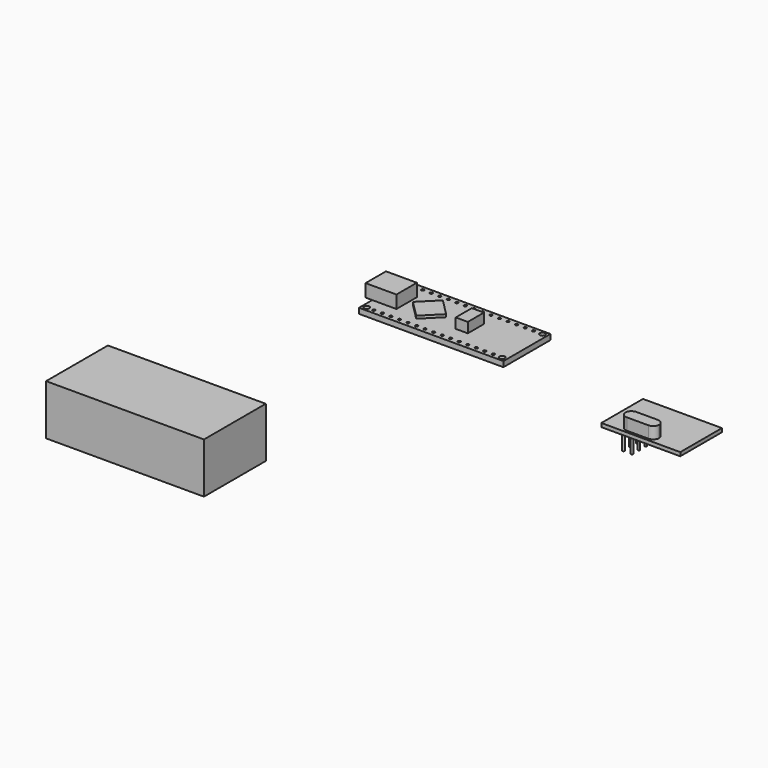
from build123d import *

# Parameters (mm, degrees)
F0_W         = 43
F0_H         = 17.5
F1_DEPTH     = 1.6
F2_R         = 0.8
F3_DEPTH     = 1.6
F4_R         = 0.4
F5_DEPTH     = 1.6
F6_W         = 9.2
F6_H         = 7.6
F7_DEPTH     = 3.8
F9_DEPTH     = 0.8
F10_W        = 3.6
F10_H        = 6
F11_DEPTH    = 3
F12_W        = 23.5
F12_H        = 15.5
F13_DEPTH    = 1.1
F14_W        = 10
F14_H        = 3.5
F15_DEPTH    = 3.5
F16_T1_DEPTH = 8
F17_W        = 2.54
F17_H        = 2.4
F17_H_2      = 0.14
F17_H_3      = 2.54
F18_DEPTH    = 2.6
F19_R        = 0.3
F20_DEPTH    = 5.7
F21_W        = 47
F21_H        = 23
F22_DEPTH    = 15


# Not quite as in the source:
# - a fillet or chamfer that OpenCascade refuses, or shapes differently, is made with other operations: its cross-section is extruded or revolved along the edge and cut away or added


with BuildPart() as f1:
    # F0 (on Top) → F1 (new body)
    with BuildSketch(Plane.XY):
        with Locations((-32.1257647276, 51.5529857576)):
            Rectangle(F0_W, F0_H)
    extrude(amount=F1_DEPTH)

    # F2 (on face) → F3 (cut, through all)
    with BuildSketch(Plane.XY.offset(1.6)):
        with Locations((-52.312482166, 59.0704187174)):
            Circle(F2_R)
        with Locations((-12.012482166, 59.0704187174)):
            Circle(F2_R)
        with Locations((-52.312482166, 44.0704187174)):
            Circle(F2_R)
        with Locations((-12.012482166, 44.0704187174)):
            Circle(F2_R)
    extrude(amount=-F3_DEPTH, mode=Mode.SUBTRACT)

    # F4 (on face) → F5 (cut, through all)
    with BuildSketch(Plane.XY.offset(1.6)):
        with Locations((-50.1963980496, 59.0704187174)):
            Circle(F4_R)
        with Locations((-47.6563980496, 59.0704187174)):
            Circle(F4_R)
        with Locations((-45.1163980496, 59.0704187174)):
            Circle(F4_R)
        with Locations((-42.5763980496, 59.0704187174)):
            Circle(F4_R)
        with Locations((-40.0363980496, 59.0704187174)):
            Circle(F4_R)
        with Locations((-37.4963980496, 59.0704187174)):
            Circle(F4_R)
        with Locations((-34.9563980496, 59.0704187174)):
            Circle(F4_R)
        with Locations((-32.4163980496, 59.0704187174)):
            Circle(F4_R)
        with Locations((-29.8763980496, 59.0704187174)):
            Circle(F4_R)
        with Locations((-27.3363980496, 59.0704187174)):
            Circle(F4_R)
        with Locations((-24.7963980496, 59.0704187174)):
            Circle(F4_R)
        with Locations((-22.2563980496, 59.0704187174)):
            Circle(F4_R)
        with Locations((-19.7163980496, 59.0704187174)):
            Circle(F4_R)
        with Locations((-17.1763980496, 59.0704187174)):
            Circle(F4_R)
        with Locations((-14.6363980496, 59.0704187174)):
            Circle(F4_R)
        with Locations((-50.1963980496, 44.0704187174)):
            Circle(F4_R)
        with Locations((-47.6563980496, 44.0704187174)):
            Circle(F4_R)
        with Locations((-45.1163980496, 44.0704187174)):
            Circle(F4_R)
        with Locations((-42.5763980496, 44.0704187174)):
            Circle(F4_R)
        with Locations((-40.0363980496, 44.0704187174)):
            Circle(F4_R)
        with Locations((-37.4963980496, 44.0704187174)):
            Circle(F4_R)
        with Locations((-34.9563980496, 44.0704187174)):
            Circle(F4_R)
        with Locations((-32.4163980496, 44.0704187174)):
            Circle(F4_R)
        with Locations((-29.8763980496, 44.0704187174)):
            Circle(F4_R)
        with Locations((-27.3363980496, 44.0704187174)):
            Circle(F4_R)
        with Locations((-24.7963980496, 44.0704187174)):
            Circle(F4_R)
        with Locations((-22.2563980496, 44.0704187174)):
            Circle(F4_R)
        with Locations((-19.7163980496, 44.0704187174)):
            Circle(F4_R)
        with Locations((-17.1763980496, 44.0704187174)):
            Circle(F4_R)
        with Locations((-14.6363980496, 44.0704187174)):
            Circle(F4_R)
    extrude(amount=-F5_DEPTH, mode=Mode.SUBTRACT)

    # F6 (on face) → F7 (join)
    with BuildSketch(Plane.XY.offset(1.6)):
        with Locations((-51.0257647276, 51.5529857576)):
            Rectangle(F6_W, F6_H)
    extrude(amount=F7_DEPTH)

    # F8 (on face) → F9 (join)
    with BuildSketch(Plane.XY.offset(1.6)):
        Polygon((-34.8264250206, 51.7515327083), (-39.7761724889, 56.7012801766), (-44.7259199572, 51.7515327083), (-39.7761724889, 46.80178524), align=None)
    extrude(amount=F9_DEPTH)

    # F10 (on face) → F11 (join)
    with BuildSketch(Plane.XY.offset(1.6)):
        with Locations((-27.622032243, 51.5529857576)):
            Rectangle(F10_W, F10_H)
    extrude(amount=F11_DEPTH)


with BuildPart() as f13:
    # F12 (on Top) → F13 (new body)
    with BuildSketch(Plane.XY):
        with Locations((37.7514823973, 41.2155307233)):
            Rectangle(F12_W, F12_H)
    extrude(amount=F13_DEPTH)

    # F14 (on face) → F15 (join)
    with BuildSketch(Plane.XY.offset(1.1)):
        with Locations((36.2846133113, 35.8788484633)):
            Rectangle(F14_W, F14_H)
    extrude(amount=F15_DEPTH)

    # F16: fillet of radius 1.8 on 4 edges, made by hand

    # F16_s2 → F16_t1 (cut)
    with BuildSketch(Plane.XY.offset(1.1)):
        with BuildLine():
            ThreePointArc((31.2846133113, 35.9288484633), (31.8118211052, 34.6560562572), (33.0846133113, 34.1288484633))
            Line((33.0846133113, 34.1288484633), (31.2846133113, 34.1288484633))
            Line((31.2846133113, 34.1288484633), (31.2846133113, 35.9288484633))
        make_face()
        with BuildLine():
            ThreePointArc((33.0846133113, 37.6288484633), (31.8118211052, 37.1016406694), (31.2846133113, 35.8288484633))
            Line((31.2846133113, 35.8288484633), (31.2846133113, 37.6288484633))
            Line((31.2846133113, 37.6288484633), (33.0846133113, 37.6288484633))
        make_face()
        with BuildLine():
            ThreePointArc((39.4846133113, 37.6288484633), (40.7574055174, 37.1016406694), (41.2846133113, 35.8288484633))
            Line((41.2846133113, 35.8288484633), (41.2846133113, 37.6288484633))
            Line((41.2846133113, 37.6288484633), (39.4846133113, 37.6288484633))
        make_face()
        with BuildLine():
            ThreePointArc((39.4846133113, 34.1288484633), (40.7574055174, 34.6560562572), (41.2846133113, 35.9288484633))
            Line((41.2846133113, 35.9288484633), (41.2846133113, 34.1288484633))
            Line((41.2846133113, 34.1288484633), (39.4846133113, 34.1288484633))
        make_face()
    extrude(amount=F16_T1_DEPTH, mode=Mode.SUBTRACT)

    # F17 (on face) → F18 (join)
    with BuildSketch(Plane(origin=(0, 0, 0), x_dir=(1, 0, 0), z_dir=(0, 0, -1))):
        with Locations((27.4714823973, -39.9455307233)):
            Rectangle(F17_W, F17_H)
        with Locations((30.0114823973, -39.9455307233)):
            Rectangle(F17_W, F17_H)
        Polygon((28.7414823973, -41.1455307233), (26.2014823973, -41.1455307233), (26.2014823973, -43.6855307233), (28.7414823973, -43.6855307233), (28.7414823973, -41.2855307233), align=None)
        with Locations((30.0114823973, -41.2155307233)):
            Rectangle(F17_W, F17_H_2)
        with Locations((27.4714823973, -44.9555307233)):
            Rectangle(F17_W, F17_H_3)
        with Locations((30.0114823973, -42.4855307233)):
            Rectangle(F17_W, F17_H)
        with Locations((30.0114823973, -44.9555307233)):
            Rectangle(F17_W, F17_H_3)
        with Locations((27.4714823973, -47.4955307233)):
            Rectangle(F17_W, F17_H_3)
        with Locations((30.0114823973, -47.4955307233)):
            Rectangle(F17_W, F17_H_3)
    extrude(amount=F18_DEPTH)

    # F19 (on face) → F20 (join)
    with BuildSketch(Plane(origin=(0, 0, -2.6), x_dir=(1, 0, 0), z_dir=(0, 0, -1))):
        with Locations((27.4714823973, -47.4955307233)):
            Circle(F19_R)
        with Locations((27.4714823973, -44.9555307233)):
            Circle(F19_R)
        with Locations((27.4714823973, -42.4155307233)):
            Circle(F19_R)
        with Locations((27.4714823973, -39.8755307233)):
            Circle(F19_R)
        with Locations((30.0114823973, -47.4955307233)):
            Circle(F19_R)
        with Locations((30.0114823973, -44.9555307233)):
            Circle(F19_R)
        with Locations((30.0114823973, -42.4155307233)):
            Circle(F19_R)
        with Locations((30.0114823973, -39.8755307233)):
            Circle(F19_R)
    extrude(amount=F20_DEPTH)


with BuildPart() as f22:
    # F21 (on Top) → F22 (new body)
    with BuildSketch(Plane.XY):
        with Locations((-47.7691207677, -40.0789575875)):
            Rectangle(F21_W, F21_H)
    extrude(amount=F22_DEPTH)


solid = Compound([f1.part, f13.part, f22.part])
